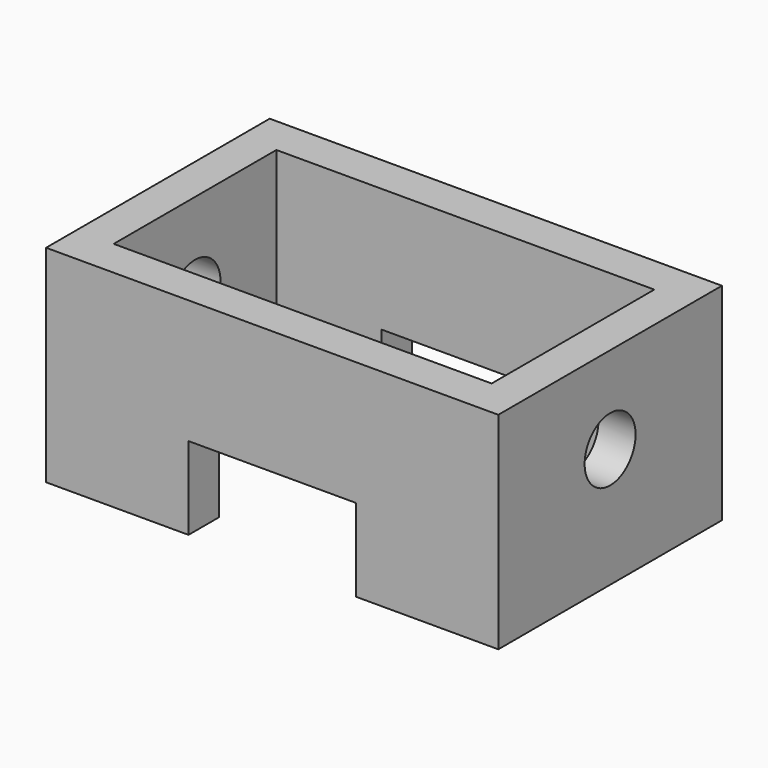
from build123d import *

# Parameters (mm, degrees)
F0_W     = 139.073908329
F0_H     = 85.957378149
F0_W_2   = 116.2280887365
F0_H_2   = 62.5404193997
F1_DEPTH = 63.5
F2_W     = 51.4795817435
F2_H     = 101.4539152384
F3_DEPTH = 25.4
F4_DEPTH = 25.4
F5_R     = 9.7930895965
F6_DEPTH = 69.5379541645


# Not quite as in the source:
# - a pattern or mirror of a feature is missing from the dataset's text; its kind, count and spacing are read off the source's solid


with BuildPart() as f1:
    # F0 (on Top) → F1 (new body)
    with BuildSketch(Plane.XY):
        Rectangle(F0_W, F0_H)
        Rectangle(F0_W_2, F0_H_2, mode=Mode.SUBTRACT)
    extrude(amount=F1_DEPTH)

    # F2 (on Top) → F3 (join)
    with BuildSketch(Plane.XY):
        Rectangle(F2_W, F2_H)
    extrude(amount=F3_DEPTH)

    # F2 (on Top) → F4 (cut)
    with BuildSketch(Plane.XY):
        Rectangle(F2_W, F2_H)
    extrude(amount=F4_DEPTH, mode=Mode.SUBTRACT)

    # F5 (on Right) → F6 (cut, through all)
    with BuildSketch(Plane.YZ):
        with Locations((0, 36.6961322725)):
            Circle(F5_R)
    f6 = extrude(amount=-F6_DEPTH, mode=Mode.SUBTRACT)

    # F6_copies: F6 across plane
    add(f6.mirror(Plane(origin=(0, 0, 0), x_dir=(0, 0, 1), z_dir=(1, 0, 0))), mode=Mode.SUBTRACT)


solid = f1.part
